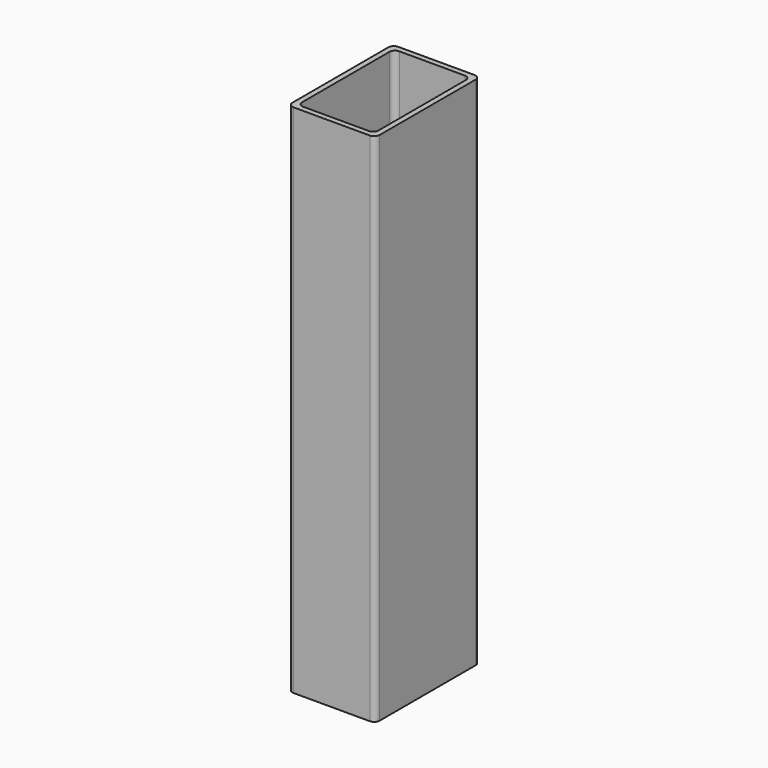
from build123d import *

# Parameters (mm, degrees)
F0_W     = 50.8
F0_H     = 76.2
F0_W_2   = 44.45
F0_H_2   = 69.85
F2_DEPTH = 300
F3_R     = 3.175


# Not quite as in the source:
# - a variable given as a bare number and used for a length is read in inches; the dataset says mm whatever the document's units were


with BuildPart() as f2:
    # F0 (on Top) → F2 (new body)
    with BuildSketch(Plane.XY):
        Rectangle(F0_W, F0_H)
        Rectangle(F0_W_2, F0_H_2, mode=Mode.SUBTRACT)
    extrude(amount=F2_DEPTH)

    # F3
    f3_edges = [f2.edges().sort_by_distance(p)[0] for p in [
        (-22.225, 34.925, 150),
        (22.225, 34.925, 150),
        (22.225, -34.925, 150),
        (-22.225, -34.925, 150),
        (25.4, 38.1, 150),
        (-25.4, 38.1, 150),
        (25.4, -38.1, 150),
        (-25.4, -38.1, 150),
    ]]
    fillet(f3_edges, radius=F3_R)


solid = f2.part
